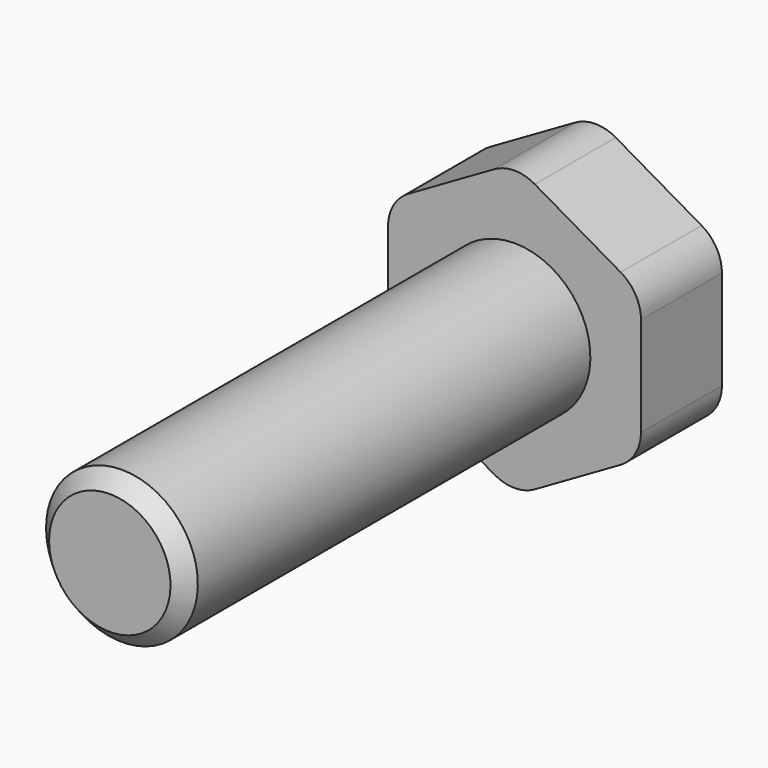
from build123d import *

# Parameters (mm, degrees)
F2_R     = 8.2875
F3_DEPTH = 25


# Not quite as in the source:
# - a feature names something its author has since deleted; it is built from what else it names


with BuildPart() as f1:
    # F0 (on Right) → F1 (revolve)
    with BuildSketch(Plane.YZ):
        Polygon((0, 8.2875), (0, 3), (-19.4, 3), (-20, 2.4), (-20, 0), (4, 0), (4, 8.2875), align=None)
    revolve(axis=Axis((0, -8, 0), (0, -1, 0)))

    # F2 (on face) → F3 (cut)
    with BuildSketch(Plane(origin=(0, 4, 0), x_dir=(-1, 0, 0), z_dir=(0, 1, 0))):
        Circle(F2_R)
        with BuildLine():
            ThreePointArc((0.803173326, -5.3097903559), (0, -5.525), (-0.803173326, -5.3097903559))
            Line((-0.803173326, -5.3097903559), (-4.196826674, -3.3504636819))
            ThreePointArc((-4.196826674, -3.3504636819), (-4.7847903559, -2.7625), (-5, -1.959326674))
            Line((-5, -1.959326674), (-5, 1.959326674))
            ThreePointArc((-5, 1.959326674), (-4.7847903559, 2.7625), (-4.196826674, 3.3504636819))
            Line((-4.196826674, 3.3504636819), (-0.803173326, 5.3097903559))
            ThreePointArc((-0.803173326, 5.3097903559), (0, 5.525), (0.803173326, 5.3097903559))
            Line((0.803173326, 5.3097903559), (4.196826674, 3.3504636819))
            ThreePointArc((4.196826674, 3.3504636819), (4.7847903559, 2.7625), (5, 1.959326674))
            Line((5, 1.959326674), (5, -1.959326674))
            ThreePointArc((5, -1.959326674), (4.7847903559, -2.7625), (4.196826674, -3.3504636819))
            Line((4.196826674, -3.3504636819), (0.803173326, -5.3097903559))
        make_face(mode=Mode.SUBTRACT)
    extrude(amount=-F3_DEPTH, mode=Mode.SUBTRACT)


solid = f1.part
